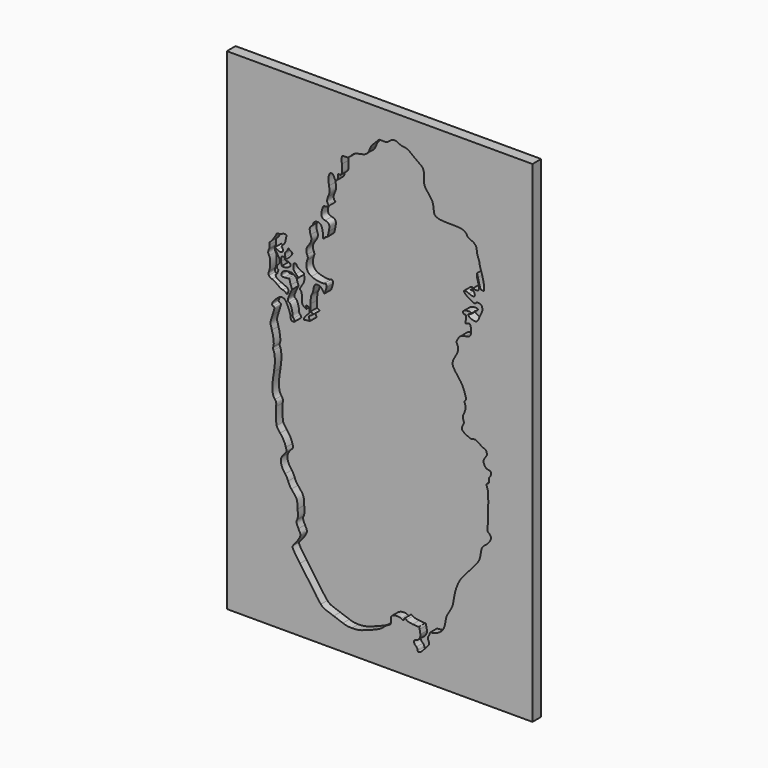
from build123d import *

# Parameters (mm, degrees)
F0_W     = 112
F0_H     = 180
F1_DEPTH = 3
F2_W     = 112
F2_H     = 180
F3_DEPTH = 1


# Not quite as in the source:
# - ends of sketch curves that miss each other by under 0.0002 mm in the source are joined


with BuildPart() as f1:
    # F0 (on Front) → F1 (new body)
    with BuildSketch(Plane.XZ):
        Rectangle(F0_W, F0_H)
        with BuildLine():
            add(Edge.make_bspline(
                [(-33.452207, 20.1281), (-33.452207, 18.937311), (-33.942265, 18.492438), (-34.505892, 19.171568)],
                knots=[0, 0, 0, 0, 1, 1, 1, 1], degree=3))
            add(Edge.make_bspline(
                [(-34.505892, 19.171568), (-34.648261, 19.343113), (-35.112361, 19.545961), (-35.537226, 19.622341)],
                knots=[0, 0, 0, 0, 1, 1, 1, 1], degree=3))
            add(Edge.make_bspline(
                [(-35.537226, 19.622341), (-35.985093, 19.702854), (-36.785926, 20.149145), (-37.44296, 20.684371)],
                knots=[0, 0, 0, 0, 1, 1, 1, 1], degree=3))
            add(Edge.make_bspline(
                [(-37.44296, 20.684371), (-38.066249, 21.192106), (-38.956872, 21.721577), (-39.42212, 21.860967)],
                knots=[0, 0, 0, 0, 1, 1, 1, 1], degree=3))
            add(Edge.make_bspline(
                [(-39.42212, 21.860967), (-39.887369, 22.00036), (-40.413552, 22.336506), (-40.591415, 22.60796)],
                knots=[0, 0, 0, 0, 1, 1, 1, 1], degree=3))
            add(Edge.make_bspline(
                [(-40.591415, 22.60796), (-40.884851, 23.055799), (-40.878115, 23.19424), (-40.518688, 24.102673)],
                knots=[0, 0, 0, 0, 1, 1, 1, 1], degree=3))
            add(Edge.make_bspline(
                [(-40.518688, 24.102673), (-39.981468, 25.46047), (-39.965306, 28.273475), (-40.490123, 29.074448)],
                knots=[0, 0, 0, 0, 1, 1, 1, 1], degree=3))
            add(Edge.make_bspline(
                [(-40.490123, 29.074448), (-40.941459, 29.763275), (-40.958652, 30.332629), (-40.551871, 31.119259)],
                knots=[0, 0, 0, 0, 1, 1, 1, 1], degree=3))
            add(Edge.make_bspline(
                [(-40.551871, 31.119259), (-40.351264, 31.507192), (-40.288878, 31.997631), (-40.373672, 32.520154)],
                knots=[0, 0, 0, 0, 1, 1, 1, 1], degree=3))
            add(Edge.make_bspline(
                [(-40.373672, 32.520154), (-40.485237, 33.207653), (-40.426908, 33.388001), (-39.97111, 33.764826)],
                knots=[0, 0, 0, 0, 1, 1, 1, 1], degree=3))
            add(Edge.make_bspline(
                [(-39.97111, 33.764826), (-39.453275, 34.19294), (-38.119119, 36.156558), (-37.838064, 36.904252)],
                knots=[0, 0, 0, 0, 1, 1, 1, 1], degree=3))
            add(Edge.make_bspline(
                [(-37.838064, 36.904252), (-37.73813, 37.170111), (-37.465273, 37.274669), (-36.871434, 37.274669)],
                knots=[0, 0, 0, 0, 1, 1, 1, 1], degree=3))
            add(Edge.make_bspline(
                [(-36.871434, 37.274669), (-36.394197, 37.274669), (-35.932527, 37.409038), (-35.78054, 37.592169)],
                knots=[0, 0, 0, 0, 1, 1, 1, 1], degree=3))
            add(Edge.make_bspline(
                [(-35.78054, 37.592169), (-35.635614, 37.766794), (-35.201315, 37.909669), (-34.81543, 37.909669)],
                knots=[0, 0, 0, 0, 1, 1, 1, 1], degree=3))
            add(Edge.make_bspline(
                [(-34.81543, 37.909669), (-34.12552, 37.909669), (-34.115723, 37.89644), (-34.227866, 37.115919)],
                knots=[0, 0, 0, 0, 1, 1, 1, 1], degree=3))
            add(Edge.make_bspline(
                [(-34.227866, 37.115919), (-34.465384, 35.462792), (-34.746487, 34.75187), (-35.370122, 34.227116)],
                knots=[0, 0, 0, 0, 1, 1, 1, 1], degree=3))
            add(Edge.make_bspline(
                [(-35.370122, 34.227116), (-35.987808, 33.707369), (-35.99809, 33.670422), (-35.666071, 33.163698)],
                knots=[0, 0, 0, 0, 1, 1, 1, 1], degree=3))
            add(Edge.make_bspline(
                [(-35.666071, 33.163698), (-34.871015, 31.950289), (-36.098201, 31.13996), (-37.504851, 31.949527)],
                knots=[0, 0, 0, 0, 1, 1, 1, 1], degree=3))
            add(Edge.make_bspline(
                [(-37.504851, 31.949527), (-37.9414, 32.200773), (-38.348154, 32.406336), (-38.408749, 32.406336)],
                knots=[0, 0, 0, 0, 1, 1, 1, 1], degree=3))
            add(Edge.make_bspline(
                [(-38.408749, 32.406336), (-38.626291, 32.406336), (-38.234714, 31.645251), (-37.438128, 30.519796)],
                knots=[0, 0, 0, 0, 1, 1, 1, 1], degree=3))
            add(Edge.make_bspline(
                [(-37.438128, 30.519796), (-36.438781, 29.10787), (-36.348556, 28.085243), (-37.156373, 27.326336)],
                knots=[0, 0, 0, 0, 1, 1, 1, 1], degree=3))
            add(Edge.make_bspline(
                [(-37.156373, 27.326336), (-37.745641, 26.772748), (-37.875697, 25.844669), (-37.364007, 25.844669)],
                knots=[0, 0, 0, 0, 1, 1, 1, 1], degree=3))
            add(Edge.make_bspline(
                [(-37.364007, 25.844669), (-37.120623, 25.844669), (-37.076294, 25.703194), (-37.181621, 25.262586)],
                knots=[0, 0, 0, 0, 1, 1, 1, 1], degree=3))
            add(Edge.make_bspline(
                [(-37.181621, 25.262586), (-37.371891, 24.46664), (-37.659904, 23.939669), (-37.904654, 23.939669)],
                knots=[0, 0, 0, 0, 1, 1, 1, 1], degree=3))
            add(Edge.make_bspline(
                [(-37.904654, 23.939669), (-38.249061, 23.939669), (-38.131257, 23.178873), (-37.730723, 22.816394)],
                knots=[0, 0, 0, 0, 1, 1, 1, 1], degree=3))
            add(Edge.make_bspline(
                [(-37.730723, 22.816394), (-37.522741, 22.628172), (-36.879803, 22.270929), (-36.301973, 22.022519)],
                knots=[0, 0, 0, 0, 1, 1, 1, 1], degree=3))
            add(Edge.make_bspline(
                [(-36.301973, 22.022519), (-33.610738, 20.865557), (-33.452207, 20.760171), (-33.452207, 20.1281)],
                knots=[0, 0, 0, 0, 1, 1, 1, 1], degree=3))
        make_face(mode=Mode.SUBTRACT)
        with BuildLine():
            add(Edge.make_bspline(
                [(-33.340422, 27.616181), (-33.616353, 27.238822), (-35.648352, 26.940163), (-35.837719, 27.249133)],
                knots=[0, 0, 0, 0, 1, 1, 1, 1], degree=3))
            add(Edge.make_bspline(
                [(-35.837719, 27.249133), (-35.89942, 27.349804), (-36.013493, 27.956044), (-36.091215, 28.596336)],
                knots=[0, 0, 0, 0, 1, 1, 1, 1], degree=3))
            add(Edge.make_bspline(
                [(-36.091215, 28.596336), (-36.274204, 30.10386), (-35.909746, 30.724602), (-35.067067, 30.340649)],
                knots=[0, 0, 0, 0, 1, 1, 1, 1], degree=3))
            add(Edge.make_bspline(
                [(-35.067067, 30.340649), (-34.706043, 30.176155), (-34.561325, 29.980284), (-34.643192, 29.766942)],
                knots=[0, 0, 0, 0, 1, 1, 1, 1], degree=3))
            add(Edge.make_bspline(
                [(-34.643192, 29.766942), (-34.738688, 29.51808), (-34.611852, 29.443002), (-34.095937, 29.443002)],
                knots=[0, 0, 0, 0, 1, 1, 1, 1], degree=3))
            add(Edge.make_bspline(
                [(-34.095937, 29.443002), (-33.144865, 29.443002), (-32.60554, 29.095631), (-32.60554, 28.483057)],
                knots=[0, 0, 0, 0, 1, 1, 1, 1], degree=3))
            add(Edge.make_bspline(
                [(-32.60554, 28.483057), (-32.60554, 28.196111), (-32.714102, 27.961336), (-32.846789, 27.961336)],
                knots=[0, 0, 0, 0, 1, 1, 1, 1], degree=3))
            add(Edge.make_bspline(
                [(-32.846789, 27.961336), (-32.979476, 27.961336), (-33.201611, 27.806015), (-33.340422, 27.616181)],
                knots=[0, 0, 0, 0, 1, 1, 1, 1], degree=3))
        make_face(mode=Mode.SUBTRACT)
        with BuildLine():
            add(Edge.make_bspline(
                [(-32.939588, 31.083419), (-34.007659, 29.963927), (-34.186452, 29.895773), (-34.503093, 30.487421)],
                knots=[0, 0, 0, 0, 1, 1, 1, 1], degree=3))
            add(Edge.make_bspline(
                [(-34.503093, 30.487421), (-34.871546, 31.175883), (-34.750485, 31.973967), (-34.19304, 32.531412)],
                knots=[0, 0, 0, 0, 1, 1, 1, 1], degree=3))
            add(Edge.make_bspline(
                [(-34.19304, 32.531412), (-33.901999, 32.822454), (-33.663874, 33.199123), (-33.663874, 33.368456)],
                knots=[0, 0, 0, 0, 1, 1, 1, 1], degree=3))
            add(Edge.make_bspline(
                [(-33.663874, 33.368456), (-33.663874, 33.537789), (-33.568624, 33.676336), (-33.452207, 33.676336)],
                knots=[0, 0, 0, 0, 1, 1, 1, 1], degree=3))
            add(Edge.make_bspline(
                [(-33.452207, 33.676336), (-33.33579, 33.676336), (-33.24054, 33.601969), (-33.24054, 33.511077)],
                knots=[0, 0, 0, 0, 1, 1, 1, 1], degree=3))
            add(Edge.make_bspline(
                [(-33.24054, 33.511077), (-33.24054, 33.420182), (-32.95479, 33.237955), (-32.60554, 33.106127)],
                knots=[0, 0, 0, 0, 1, 1, 1, 1], degree=3))
            add(Edge.make_bspline(
                [(-32.60554, 33.106127), (-31.721987, 32.772625), (-31.804468, 32.273189), (-32.939588, 31.083419)],
                knots=[0, 0, 0, 0, 1, 1, 1, 1], degree=3))
        make_face(mode=Mode.SUBTRACT)
        with BuildLine():
            add(Edge.make_bspline(
                [(-33.181515, 16.37951), (-33.856509, 16.687056), (-33.794526, 17.270613), (-32.88299, 19.190049)],
                knots=[0, 0, 0, 0, 1, 1, 1, 1], degree=3))
            Line((-32.88299, 19.190049), (-32.102106, 20.834368))
            Line((-32.102106, 20.834368), (-32.56549, 22.162106))
            add(Edge.make_bspline(
                [(-32.56549, 22.162106), (-32.820351, 22.892361), (-33.028874, 23.645098), (-33.028874, 23.834852)],
                knots=[0, 0, 0, 0, 1, 1, 1, 1], degree=3))
            add(Edge.make_bspline(
                [(-33.028874, 23.834852), (-33.028874, 24.101586), (-33.136928, 24.141533), (-33.505124, 24.010929)],
                knots=[0, 0, 0, 0, 1, 1, 1, 1], degree=3))
            add(Edge.make_bspline(
                [(-33.505124, 24.010929), (-33.767061, 23.918015), (-34.409999, 23.840159), (-34.933874, 23.837916)],
                knots=[0, 0, 0, 0, 1, 1, 1, 1], degree=3))
            add(Edge.make_bspline(
                [(-34.933874, 23.837916), (-35.841877, 23.834026), (-35.889325, 23.864003), (-35.949561, 24.479652)],
                knots=[0, 0, 0, 0, 1, 1, 1, 1], degree=3))
            add(Edge.make_bspline(
                [(-35.949561, 24.479652), (-36.054367, 25.550836), (-34.784788, 26.268002), (-32.783695, 26.268002)],
                knots=[0, 0, 0, 0, 1, 1, 1, 1], degree=3))
            add(Edge.make_bspline(
                [(-32.783695, 26.268002), (-31.934397, 26.268002), (-31.641586, 26.1596), (-31.104508, 25.646337)],
                knots=[0, 0, 0, 0, 1, 1, 1, 1], degree=3))
            add(Edge.make_bspline(
                [(-31.104508, 25.646337), (-30.746726, 25.304422), (-30.318968, 25.076488), (-30.153934, 25.139819)],
                knots=[0, 0, 0, 0, 1, 1, 1, 1], degree=3))
            add(Edge.make_bspline(
                [(-30.153934, 25.139819), (-29.704821, 25.312158), (-29.774591, 25.46967), (-30.70054, 26.373836)],
                knots=[0, 0, 0, 0, 1, 1, 1, 1], degree=3))
            add(Edge.make_bspline(
                [(-30.70054, 26.373836), (-31.495874, 27.150459), (-31.547207, 27.27498), (-31.547207, 28.427627)],
                knots=[0, 0, 0, 0, 1, 1, 1, 1], degree=3))
            add(Edge.make_bspline(
                [(-31.547207, 28.427627), (-31.547207, 29.59536), (-31.52163, 29.654669), (-31.01804, 29.654669)],
                knots=[0, 0, 0, 0, 1, 1, 1, 1], degree=3))
            add(Edge.make_bspline(
                [(-31.01804, 29.654669), (-30.703175, 29.654669), (-30.488874, 29.533506), (-30.488874, 29.355481)],
                knots=[0, 0, 0, 0, 1, 1, 1, 1], degree=3))
            add(Edge.make_bspline(
                [(-30.488874, 29.355481), (-30.488874, 28.942654), (-28.818079, 27.749669), (-28.239906, 27.749669)],
                knots=[0, 0, 0, 0, 1, 1, 1, 1], degree=3))
            add(Edge.make_bspline(
                [(-28.239906, 27.749669), (-27.826624, 27.749669), (-27.749631, 27.605302), (-27.623187, 26.593281)],
                knots=[0, 0, 0, 0, 1, 1, 1, 1], degree=3))
            add(Edge.make_bspline(
                [(-27.623187, 26.593281), (-27.456287, 25.257458), (-27.655596, 24.548041), (-28.571998, 23.216097)],
                knots=[0, 0, 0, 0, 1, 1, 1, 1], degree=3))
            add(Edge.make_bspline(
                [(-28.571998, 23.216097), (-29.211875, 22.286068), (-29.401763, 21.611336), (-29.023622, 21.611336)],
                knots=[0, 0, 0, 0, 1, 1, 1, 1], degree=3))
            add(Edge.make_bspline(
                [(-29.023622, 21.611336), (-28.661322, 21.611336), (-28.350372, 20.184647), (-28.485856, 19.143974)],
                knots=[0, 0, 0, 0, 1, 1, 1, 1], degree=3))
            add(Edge.make_bspline(
                [(-28.485856, 19.143974), (-28.655825, 17.838422), (-28.355406, 17.06631), (-27.506697, 16.627424)],
                knots=[0, 0, 0, 0, 1, 1, 1, 1], degree=3))
            Line((-27.506697, 16.627424), (-26.834667, 16.279905))
            Line((-26.834667, 16.279905), (-26.97247, 16.828955))
            add(Edge.make_bspline(
                [(-26.97247, 16.828955), (-27.09716, 17.32576), (-27.051623, 17.378002), (-26.493886, 17.378002)],
                knots=[0, 0, 0, 0, 1, 1, 1, 1], degree=3))
            add(Edge.make_bspline(
                [(-26.493886, 17.378002), (-25.814757, 17.378002), (-25.6215, 17.082016), (-25.618818, 16.037774)],
                knots=[0, 0, 0, 0, 1, 1, 1, 1], degree=3))
            add(Edge.make_bspline(
                [(-25.618818, 16.037774), (-25.617469, 15.509523), (-25.818313, 15.18744), (-26.564986, 14.520502)],
                knots=[0, 0, 0, 0, 1, 1, 1, 1], degree=3))
            add(Edge.make_bspline(
                [(-26.564986, 14.520502), (-27.088954, 14.052486), (-27.576987, 13.398825), (-27.65623, 13.05891)],
                knots=[0, 0, 0, 0, 1, 1, 1, 1], degree=3))
            add(Edge.make_bspline(
                [(-27.65623, 13.05891), (-27.789069, 12.489095), (-27.762358, 12.453945), (-27.292147, 12.57977)],
                knots=[0, 0, 0, 0, 1, 1, 1, 1], degree=3))
            add(Edge.make_bspline(
                [(-27.292147, 12.57977), (-27.013055, 12.654452), (-26.471793, 12.716856), (-26.089343, 12.718446)],
                knots=[0, 0, 0, 0, 1, 1, 1, 1], degree=3))
            add(Edge.make_bspline(
                [(-26.089343, 12.718446), (-25.467765, 12.721092), (-25.41723, 12.764778), (-25.613093, 13.130755)],
                knots=[0, 0, 0, 0, 1, 1, 1, 1], degree=3))
            add(Edge.make_bspline(
                [(-25.613093, 13.130755), (-26.016484, 13.884497), (-25.882158, 14.605735), (-25.311723, 14.748904)],
                knots=[0, 0, 0, 0, 1, 1, 1, 1], degree=3))
            add(Edge.make_bspline(
                [(-25.311723, 14.748904), (-25.025456, 14.820751), (-24.681728, 15.01149), (-24.547883, 15.172761)],
                knots=[0, 0, 0, 0, 1, 1, 1, 1], degree=3))
            add(Edge.make_bspline(
                [(-24.547883, 15.172761), (-24.354366, 15.405936), (-24.416942, 15.508726), (-24.85344, 15.674684)],
                knots=[0, 0, 0, 0, 1, 1, 1, 1], degree=3))
            Line((-24.85344, 15.674684), (-25.402351, 15.883379))
            Line((-25.402351, 15.883379), (-25.337298, 18.401704))
            add(Edge.make_bspline(
                [(-25.337298, 18.401704), (-25.283362, 20.489637), (-25.197538, 21.046649), (-24.835122, 21.660895)],
                knots=[0, 0, 0, 0, 1, 1, 1, 1], degree=3))
            add(Edge.make_bspline(
                [(-24.835122, 21.660895), (-24.594705, 22.068374), (-24.329432, 22.91448), (-24.245626, 23.541132)],
                knots=[0, 0, 0, 0, 1, 1, 1, 1], degree=3))
            add(Edge.make_bspline(
                [(-24.245626, 23.541132), (-24.053642, 24.976677), (-23.674132, 25.421336), (-22.640895, 25.421336)],
                knots=[0, 0, 0, 0, 1, 1, 1, 1], degree=3))
            add(Edge.make_bspline(
                [(-22.640895, 25.421336), (-21.966808, 25.421336), (-21.726439, 25.284546), (-21.086201, 24.536569)],
                knots=[0, 0, 0, 0, 1, 1, 1, 1], degree=3))
            add(Edge.make_bspline(
                [(-21.086201, 24.536569), (-20.669671, 24.049947), (-20.323552, 23.549885), (-20.317048, 23.425319)],
                knots=[0, 0, 0, 0, 1, 1, 1, 1], degree=3))
            add(Edge.make_bspline(
                [(-20.317048, 23.425319), (-20.291121, 22.928799), (-19.505283, 25.146547), (-19.497276, 25.738836)],
                knots=[0, 0, 0, 0, 1, 1, 1, 1], degree=3))
            add(Edge.make_bspline(
                [(-19.497276, 25.738836), (-19.484513, 26.683165), (-19.747962, 27.005002), (-20.267936, 26.680271)],
                knots=[0, 0, 0, 0, 1, 1, 1, 1], degree=3))
            add(Edge.make_bspline(
                [(-20.267936, 26.680271), (-20.841746, 26.321922), (-23.700708, 26.748536), (-24.985541, 27.384234)],
                knots=[0, 0, 0, 0, 1, 1, 1, 1], degree=3))
            add(Edge.make_bspline(
                [(-24.985541, 27.384234), (-26.691258, 28.228173), (-27.267401, 29.9549), (-26.547871, 32.066603)],
                knots=[0, 0, 0, 0, 1, 1, 1, 1], degree=3))
            add(Edge.make_bspline(
                [(-26.547871, 32.066603), (-26.227972, 33.005458), (-26.22989, 33.127032), (-26.576744, 33.896215)],
                knots=[0, 0, 0, 0, 1, 1, 1, 1], degree=3))
            add(Edge.make_bspline(
                [(-26.576744, 33.896215), (-27.035529, 34.91362), (-26.897942, 35.994083), (-26.191194, 36.923929)],
                knots=[0, 0, 0, 0, 1, 1, 1, 1], degree=3))
            add(Edge.make_bspline(
                [(-26.191194, 36.923929), (-24.961255, 38.542121), (-24.755625, 39.424372), (-25.303041, 40.734522)],
                knots=[0, 0, 0, 0, 1, 1, 1, 1], degree=3))
            add(Edge.make_bspline(
                [(-25.303041, 40.734522), (-25.477666, 41.152458), (-25.620541, 41.871979), (-25.620541, 42.33346)],
                knots=[0, 0, 0, 0, 1, 1, 1, 1], degree=3))
            add(Edge.make_bspline(
                [(-25.620541, 42.33346), (-25.620541, 43.024147), (-25.508258, 43.252464), (-24.985541, 43.624672)],
                knots=[0, 0, 0, 0, 1, 1, 1, 1], degree=3))
            add(Edge.make_bspline(
                [(-24.985541, 43.624672), (-24.636291, 43.873359), (-24.350541, 44.257134), (-24.350541, 44.477506)],
                knots=[0, 0, 0, 0, 1, 1, 1, 1], degree=3))
            add(Edge.make_bspline(
                [(-24.350541, 44.477506), (-24.350541, 45.594248), (-22.431199, 46.16264), (-21.615768, 45.287374)],
                knots=[0, 0, 0, 0, 1, 1, 1, 1], degree=3))
            add(Edge.make_bspline(
                [(-21.615768, 45.287374), (-21.109145, 44.743579), (-20.662783, 42.776066), (-20.822605, 41.791199)],
                knots=[0, 0, 0, 0, 1, 1, 1, 1], degree=3))
            add(Edge.make_bspline(
                [(-20.822605, 41.791199), (-20.954781, 40.976693), (-20.499399, 40.793873), (-20.117207, 41.508005)],
                knots=[0, 0, 0, 0, 1, 1, 1, 1], degree=3))
            add(Edge.make_bspline(
                [(-20.117207, 41.508005), (-19.992599, 41.740838), (-19.705312, 41.931338), (-19.478793, 41.931338)],
                knots=[0, 0, 0, 0, 1, 1, 1, 1], degree=3))
            add(Edge.make_bspline(
                [(-19.478793, 41.931338), (-19.198062, 41.931338), (-19.030888, 42.116655), (-18.953701, 42.513422)],
                knots=[0, 0, 0, 0, 1, 1, 1, 1], degree=3))
            add(Edge.make_bspline(
                [(-18.953701, 42.513422), (-18.89142, 42.833567), (-18.746731, 43.501683), (-18.632169, 43.998126)],
                knots=[0, 0, 0, 0, 1, 1, 1, 1], degree=3))
            add(Edge.make_bspline(
                [(-18.632169, 43.998126), (-18.149076, 46.091551), (-18.464465, 46.832284), (-19.952374, 47.09881)],
                knots=[0, 0, 0, 0, 1, 1, 1, 1], degree=3))
            add(Edge.make_bspline(
                [(-19.952374, 47.09881), (-21.372442, 47.353185), (-21.67856, 48.313191), (-21.020685, 50.449112)],
                knots=[0, 0, 0, 0, 1, 1, 1, 1], degree=3))
            add(Edge.make_bspline(
                [(-21.020685, 50.449112), (-20.672024, 51.581108), (-20.602006, 51.66451), (-19.998913, 51.666195)],
                knots=[0, 0, 0, 0, 1, 1, 1, 1], degree=3))
            add(Edge.make_bspline(
                [(-19.998913, 51.666195), (-19.64281, 51.667254), (-19.167823, 51.802276), (-18.943389, 51.966386)],
                knots=[0, 0, 0, 0, 1, 1, 1, 1], degree=3))
            add(Edge.make_bspline(
                [(-18.943389, 51.966386), (-18.555059, 52.250342), (-18.553103, 52.28441), (-18.902935, 52.670969)],
                knots=[0, 0, 0, 0, 1, 1, 1, 1], degree=3))
            add(Edge.make_bspline(
                [(-18.902935, 52.670969), (-19.361289, 53.177445), (-19.371368, 53.987205), (-18.932029, 55.008553)],
                knots=[0, 0, 0, 0, 1, 1, 1, 1], degree=3))
            add(Edge.make_bspline(
                [(-18.932029, 55.008553), (-18.259801, 56.571305), (-18.220416, 56.95618), (-18.553202, 58.71048)],
                knots=[0, 0, 0, 0, 1, 1, 1, 1], degree=3))
            add(Edge.make_bspline(
                [(-18.553202, 58.71048), (-19.053729, 61.349042), (-18.663629, 63.098004), (-17.574581, 63.098004)],
                knots=[0, 0, 0, 0, 1, 1, 1, 1], degree=3))
            add(Edge.make_bspline(
                [(-17.574581, 63.098004), (-17.130381, 63.098004), (-16.932486, 62.855999), (-16.624707, 61.936416)],
                knots=[0, 0, 0, 0, 1, 1, 1, 1], degree=3))
            add(Edge.make_bspline(
                [(-16.624707, 61.936416), (-16.185222, 60.623311), (-15.248874, 61.364218), (-15.248874, 63.025077)],
                knots=[0, 0, 0, 0, 1, 1, 1, 1], degree=3))
            add(Edge.make_bspline(
                [(-15.248874, 63.025077), (-15.248874, 63.724734), (-15.210609, 63.769293), (-14.716325, 63.645236)],
                knots=[0, 0, 0, 0, 1, 1, 1, 1], degree=3))
            add(Edge.make_bspline(
                [(-14.716325, 63.645236), (-13.8828, 63.436035), (-13.698338, 64.212786), (-13.859917, 67.251448)],
                knots=[0, 0, 0, 0, 1, 1, 1, 1], degree=3))
            add(Edge.make_bspline(
                [(-13.859917, 67.251448), (-14.013915, 70.147494), (-14.056947, 70.07356), (-12.213489, 70.080114)],
                knots=[0, 0, 0, 0, 1, 1, 1, 1], degree=3))
            add(Edge.make_bspline(
                [(-12.213489, 70.080114), (-11.518957, 70.082575), (-11.254887, 70.234186), (-10.399825, 71.12133)],
                knots=[0, 0, 0, 0, 1, 1, 1, 1], degree=3))
            add(Edge.make_bspline(
                [(-10.399825, 71.12133), (-9.375891, 72.183684), (-9.027265, 72.337554), (-6.515171, 72.835877)],
                knots=[0, 0, 0, 0, 1, 1, 1, 1], degree=3))
            add(Edge.make_bspline(
                [(-6.515171, 72.835877), (-4.934002, 73.149533), (-4.211332, 73.775078), (-3.703224, 75.269907)],
                knots=[0, 0, 0, 0, 1, 1, 1, 1], degree=3))
            add(Edge.make_bspline(
                [(-3.703224, 75.269907), (-3.384936, 76.206291), (-2.963105, 76.802249), (-1.745516, 78.035737)],
                knots=[0, 0, 0, 0, 1, 1, 1, 1], degree=3))
            Line((-1.745516, 78.035737), (-0.193515, 79.608005))
            Line((-0.193515, 79.608005), (1.274028, 79.608005))
            add(Edge.make_bspline(
                [(1.274028, 79.608005), (2.657944, 79.608005), (2.788984, 79.650838), (3.573572, 80.359667)],
                knots=[0, 0, 0, 0, 1, 1, 1, 1], degree=3))
            add(Edge.make_bspline(
                [(3.573572, 80.359667), (4.717466, 81.393106), (5.622754, 81.514468), (6.844933, 80.798222)],
                knots=[0, 0, 0, 0, 1, 1, 1, 1], degree=3))
            add(Edge.make_bspline(
                [(6.844933, 80.798222), (7.393068, 80.476995), (8.113838, 80.243005), (8.5552, 80.243005)],
                knots=[0, 0, 0, 0, 1, 1, 1, 1], degree=3))
            add(Edge.make_bspline(
                [(8.5552, 80.243005), (9.646529, 80.243005), (10.657992, 79.759654), (12.025824, 78.584484)],
                knots=[0, 0, 0, 0, 1, 1, 1, 1], degree=3))
            add(Edge.make_bspline(
                [(12.025824, 78.584484), (12.682782, 78.020062), (13.763409, 77.213935), (14.427222, 76.793091)],
                knots=[0, 0, 0, 0, 1, 1, 1, 1], degree=3))
            add(Edge.make_bspline(
                [(14.427222, 76.793091), (16.074841, 75.748531), (16.306735, 75.227319), (16.257758, 72.678687)],
                knots=[0, 0, 0, 0, 1, 1, 1, 1], degree=3))
            add(Edge.make_bspline(
                [(16.257758, 72.678687), (16.212196, 70.307789), (16.302787, 70.061232), (17.989212, 67.966338)],
                knots=[0, 0, 0, 0, 1, 1, 1, 1], degree=3))
            add(Edge.make_bspline(
                [(17.989212, 67.966338), (19.344001, 66.283404), (19.583327, 65.731341), (19.778539, 63.838838)],
                knots=[0, 0, 0, 0, 1, 1, 1, 1], degree=3))
            add(Edge.make_bspline(
                [(19.778539, 63.838838), (19.970981, 61.973202), (20.093107, 61.754361), (21.204535, 61.283582)],
                knots=[0, 0, 0, 0, 1, 1, 1, 1], degree=3))
            add(Edge.make_bspline(
                [(21.204535, 61.283582), (21.954454, 60.965929), (22.770757, 60.893977), (25.949027, 60.865383)],
                knots=[0, 0, 0, 0, 1, 1, 1, 1], degree=3))
            add(Edge.make_bspline(
                [(25.949027, 60.865383), (29.468866, 60.833716), (29.870316, 60.790883), (30.781501, 60.349786)],
                knots=[0, 0, 0, 0, 1, 1, 1, 1], degree=3))
            add(Edge.make_bspline(
                [(30.781501, 60.349786), (31.328057, 60.085202), (31.822063, 59.71425), (31.879287, 59.525448)],
                knots=[0, 0, 0, 0, 1, 1, 1, 1], degree=3))
            add(Edge.make_bspline(
                [(31.879287, 59.525448), (32.104106, 58.783721), (32.322853, 58.58271), (33.33577, 58.18706)],
                knots=[0, 0, 0, 0, 1, 1, 1, 1], degree=3))
            add(Edge.make_bspline(
                [(33.33577, 58.18706), (34.993647, 57.539487), (35.470177, 56.959313), (35.614613, 55.412567)],
                knots=[0, 0, 0, 0, 1, 1, 1, 1], degree=3))
            add(Edge.make_bspline(
                [(35.614613, 55.412567), (35.682043, 54.690491), (35.931375, 53.671631), (36.168685, 53.148436)],
                knots=[0, 0, 0, 0, 1, 1, 1, 1], degree=3))
            add(Edge.make_bspline(
                [(36.168685, 53.148436), (36.405998, 52.625241), (36.602253, 51.938806), (36.604809, 51.623026)],
                knots=[0, 0, 0, 0, 1, 1, 1, 1], degree=3))
            add(Edge.make_bspline(
                [(36.604809, 51.623026), (36.607454, 51.307248), (36.794766, 50.545248), (37.02126, 49.929692)],
                knots=[0, 0, 0, 0, 1, 1, 1, 1], degree=3))
            add(Edge.make_bspline(
                [(37.02126, 49.929692), (37.701472, 48.081012), (38.302791, 45.422529), (38.302791, 44.26391)],
                knots=[0, 0, 0, 0, 1, 1, 1, 1], degree=3))
            Line((38.302791, 44.26391), (38.302791, 43.174515))
            Line((38.302791, 43.174515), (37.620719, 43.240843))
            add(Edge.make_bspline(
                [(37.620719, 43.240843), (36.865548, 43.314278), (36.860634, 43.325745), (36.050819, 46.905505)],
                knots=[0, 0, 0, 0, 1, 1, 1, 1], degree=3))
            add(Edge.make_bspline(
                [(36.050819, 46.905505), (35.750316, 48.233861), (35.652496, 48.453323), (35.596982, 47.923717)],
                knots=[0, 0, 0, 0, 1, 1, 1, 1], degree=3))
            add(Edge.make_bspline(
                [(35.596982, 47.923717), (35.558059, 47.552398), (35.722315, 46.613677), (35.962001, 45.837668)],
                knots=[0, 0, 0, 0, 1, 1, 1, 1], degree=3))
            add(Edge.make_bspline(
                [(35.962001, 45.837668), (36.201687, 45.061661), (36.397791, 44.158818), (36.397791, 43.831354)],
                knots=[0, 0, 0, 0, 1, 1, 1, 1], degree=3))
            add(Edge.make_bspline(
                [(36.397791, 43.831354), (36.397791, 42.724144), (36.228383, 42.566338), (35.039766, 42.566338)],
                knots=[0, 0, 0, 0, 1, 1, 1, 1], degree=3))
            add(Edge.make_bspline(
                [(35.039766, 42.566338), (34.354088, 42.566338), (33.783697, 42.440828), (33.527829, 42.233651)],
                knots=[0, 0, 0, 0, 1, 1, 1, 1], degree=3))
            add(Edge.make_bspline(
                [(33.527829, 42.233651), (33.137129, 41.917297), (33.149665, 41.906433), (33.783183, 42.012354)],
                knots=[0, 0, 0, 0, 1, 1, 1, 1], degree=3))
            add(Edge.make_bspline(
                [(33.783183, 42.012354), (34.367045, 42.109974), (34.481239, 42.046903), (34.706873, 41.502176)],
                knots=[0, 0, 0, 0, 1, 1, 1, 1], degree=3))
            add(Edge.make_bspline(
                [(34.706873, 41.502176), (35.23492, 40.22735), (34.460601, 39.889403), (32.769655, 40.65669)],
                knots=[0, 0, 0, 0, 1, 1, 1, 1], degree=3))
            add(Edge.make_bspline(
                [(32.769655, 40.65669), (29.998089, 41.91432), (30.46157, 40.257351), (33.297202, 38.770695)],
                knots=[0, 0, 0, 0, 1, 1, 1, 1], degree=3))
            add(Edge.make_bspline(
                [(33.297202, 38.770695), (34.690344, 38.040299), (35.028802, 37.981405), (35.204335, 38.438836)],
                knots=[0, 0, 0, 0, 1, 1, 1, 1], degree=3))
            add(Edge.make_bspline(
                [(35.204335, 38.438836), (35.406691, 38.966166), (36.938718, 38.856372), (37.338289, 38.285906)],
                knots=[0, 0, 0, 0, 1, 1, 1, 1], degree=3))
            add(Edge.make_bspline(
                [(37.338289, 38.285906), (37.791523, 37.638823), (37.7511, 36.506933), (37.245542, 35.688926)],
                knots=[0, 0, 0, 0, 1, 1, 1, 1], degree=3))
            add(Edge.make_bspline(
                [(37.245542, 35.688926), (37.013307, 35.313162), (36.677424, 34.59227), (36.499137, 34.08695)],
                knots=[0, 0, 0, 0, 1, 1, 1, 1], degree=3))
            add(Edge.make_bspline(
                [(36.499137, 34.08695), (36.069821, 32.870142), (35.618122, 32.406336), (34.86239, 32.406336)],
                knots=[0, 0, 0, 0, 1, 1, 1, 1], degree=3))
            add(Edge.make_bspline(
                [(34.86239, 32.406336), (34.05989, 32.406336), (32.845161, 32.983765), (32.571344, 33.495403)],
                knots=[0, 0, 0, 0, 1, 1, 1, 1], degree=3))
            add(Edge.make_bspline(
                [(32.571344, 33.495403), (32.354717, 33.900173), (32.369877, 33.913556), (33.399143, 34.22592)],
                knots=[0, 0, 0, 0, 1, 1, 1, 1], degree=3))
            add(Edge.make_bspline(
                [(33.399143, 34.22592), (33.554343, 34.273024), (33.642232, 34.430573), (33.594448, 34.576033)],
                knots=[0, 0, 0, 0, 1, 1, 1, 1], degree=3))
            add(Edge.make_bspline(
                [(33.594448, 34.576033), (33.46648, 34.965576), (32.104778, 35.015522), (31.25804, 34.661731)],
                knots=[0, 0, 0, 0, 1, 1, 1, 1], degree=3))
            add(Edge.make_bspline(
                [(31.25804, 34.661731), (30.627017, 34.398074), (30.536886, 34.274421), (30.628062, 33.797465)],
                knots=[0, 0, 0, 0, 1, 1, 1, 1], degree=3))
            add(Edge.make_bspline(
                [(30.628062, 33.797465), (30.71026, 33.367474), (30.825113, 33.269647), (31.133003, 33.367366)],
                knots=[0, 0, 0, 0, 1, 1, 1, 1], degree=3))
            add(Edge.make_bspline(
                [(31.133003, 33.367366), (31.684157, 33.542298), (31.793453, 33.125915), (31.570156, 31.701965)],
                knots=[0, 0, 0, 0, 1, 1, 1, 1], degree=3))
            add(Edge.make_bspline(
                [(31.570156, 31.701965), (31.466603, 31.04162), (31.40345, 30.501336), (31.429818, 30.501336)],
                knots=[0, 0, 0, 0, 1, 1, 1, 1], degree=3))
            add(Edge.make_bspline(
                [(31.429818, 30.501336), (31.456197, 30.501336), (31.82438, 30.646166), (32.248031, 30.823175)],
                knots=[0, 0, 0, 0, 1, 1, 1, 1], degree=3))
            add(Edge.make_bspline(
                [(32.248031, 30.823175), (33.013098, 31.142844), (33.019921, 31.141056), (33.258078, 30.558591)],
                knots=[0, 0, 0, 0, 1, 1, 1, 1], degree=3))
            add(Edge.make_bspline(
                [(33.258078, 30.558591), (33.389954, 30.236062), (33.507403, 29.432385), (33.519071, 28.772646)],
                knots=[0, 0, 0, 0, 1, 1, 1, 1], degree=3))
            add(Edge.make_bspline(
                [(33.519071, 28.772646), (33.547924, 27.141596), (33.029259, 26.568701), (31.401537, 26.433716)],
                knots=[0, 0, 0, 0, 1, 1, 1, 1], degree=3))
            add(Edge.make_bspline(
                [(31.401537, 26.433716), (29.985315, 26.316273), (29.274292, 25.826177), (28.589444, 24.495389)],
                knots=[0, 0, 0, 0, 1, 1, 1, 1], degree=3))
            add(Edge.make_bspline(
                [(28.589444, 24.495389), (28.089736, 23.524366), (28.087514, 23.495193), (28.460479, 22.802646)],
                knots=[0, 0, 0, 0, 1, 1, 1, 1], degree=3))
            add(Edge.make_bspline(
                [(28.460479, 22.802646), (29.022483, 21.759066), (28.804731, 20.502094), (27.762614, 18.774246)],
                knots=[0, 0, 0, 0, 1, 1, 1, 1], degree=3))
            add(Edge.make_bspline(
                [(27.762614, 18.774246), (26.256489, 16.27705), (26.340499, 15.601759), (28.494726, 12.889648)],
                knots=[0, 0, 0, 0, 1, 1, 1, 1], degree=3))
            add(Edge.make_bspline(
                [(28.494726, 12.889648), (30.072807, 10.902891), (30.643966, 9.852207), (31.320466, 7.691522)],
                knots=[0, 0, 0, 0, 1, 1, 1, 1], degree=3))
            add(Edge.make_bspline(
                [(31.320466, 7.691522), (31.787826, 6.198811), (31.790546, 6.141781), (31.414213, 5.725935)],
                knots=[0, 0, 0, 0, 1, 1, 1, 1], degree=3))
            add(Edge.make_bspline(
                [(31.414213, 5.725935), (31.080113, 5.356759), (31.061322, 5.201719), (31.278045, 4.602387)],
                knots=[0, 0, 0, 0, 1, 1, 1, 1], degree=3))
            add(Edge.make_bspline(
                [(31.278045, 4.602387), (31.649494, 3.575158), (31.589113, 2.919962), (31.000291, 1.588532)],
                knots=[0, 0, 0, 0, 1, 1, 1, 1], degree=3))
            add(Edge.make_bspline(
                [(31.000291, 1.588532), (30.396784, 0.223895), (30.373416, 0.004098), (30.727693, -0.975633)],
                knots=[0, 0, 0, 0, 1, 1, 1, 1], degree=3))
            add(Edge.make_bspline(
                [(30.727693, -0.975633), (30.955542, -1.605743), (30.927311, -1.789409), (30.475447, -2.616587)],
                knots=[0, 0, 0, 0, 1, 1, 1, 1], degree=3))
            add(Edge.make_bspline(
                [(30.475447, -2.616587), (29.7633, -3.920231), (30.025357, -4.405525), (31.970409, -5.385036)],
                knots=[0, 0, 0, 0, 1, 1, 1, 1], degree=3))
            add(Edge.make_bspline(
                [(31.970409, -5.385036), (33.321475, -6.065422), (33.549887, -6.120543), (34.090428, -5.896645)],
                knots=[0, 0, 0, 0, 1, 1, 1, 1], degree=3))
            add(Edge.make_bspline(
                [(34.090428, -5.896645), (34.889285, -5.565749), (35.482369, -5.737696), (36.669999, -6.644519)],
                knots=[0, 0, 0, 0, 1, 1, 1, 1], degree=3))
            add(Edge.make_bspline(
                [(36.669999, -6.644519), (37.210189, -7.056983), (37.935872, -7.451199), (38.282632, -7.520549)],
                knots=[0, 0, 0, 0, 1, 1, 1, 1], degree=3))
            add(Edge.make_bspline(
                [(38.282632, -7.520549), (38.740107, -7.612044), (38.97457, -7.822968), (39.137112, -8.28924)],
                knots=[0, 0, 0, 0, 1, 1, 1, 1], degree=3))
            add(Edge.make_bspline(
                [(39.137112, -8.28924), (39.460068, -9.215668), (39.429982, -9.35881), (38.726124, -10.244498)],
                knots=[0, 0, 0, 0, 1, 1, 1, 1], degree=3))
            add(Edge.make_bspline(
                [(38.726124, -10.244498), (37.951628, -11.219075), (37.90378, -12.125429), (38.574131, -13.123614)],
                knots=[0, 0, 0, 0, 1, 1, 1, 1], degree=3))
            add(Edge.make_bspline(
                [(38.574131, -13.123614), (38.940865, -13.669698), (39.233402, -13.859714), (39.789363, -13.912967)],
                knots=[0, 0, 0, 0, 1, 1, 1, 1], degree=3))
            add(Edge.make_bspline(
                [(39.789363, -13.912967), (40.19209, -13.951543), (40.592402, -14.094418), (40.67895, -14.230467)],
                knots=[0, 0, 0, 0, 1, 1, 1, 1], degree=3))
            add(Edge.make_bspline(
                [(40.67895, -14.230467), (40.980395, -14.704333), (40.839756, -15.579133), (40.397833, -15.979069)],
                knots=[0, 0, 0, 0, 1, 1, 1, 1], degree=3))
            add(Edge.make_bspline(
                [(40.397833, -15.979069), (40.041643, -16.301416), (39.972642, -16.557123), (40.051959, -17.260824)],
                knots=[0, 0, 0, 0, 1, 1, 1, 1], degree=3))
            add(Edge.make_bspline(
                [(40.051959, -17.260824), (40.138488, -18.028508), (40.087588, -18.168816), (39.65025, -18.368079)],
                knots=[0, 0, 0, 0, 1, 1, 1, 1], degree=3))
            add(Edge.make_bspline(
                [(39.65025, -18.368079), (39.058729, -18.637594), (39.032609, -18.909729), (39.492834, -20.008234)],
                knots=[0, 0, 0, 0, 1, 1, 1, 1], degree=3))
            add(Edge.make_bspline(
                [(39.492834, -20.008234), (39.770995, -20.672171), (39.831842, -21.57153), (39.813212, -24.743664)],
                knots=[0, 0, 0, 0, 1, 1, 1, 1], degree=3))
            add(Edge.make_bspline(
                [(39.813212, -24.743664), (39.800565, -26.897373), (39.72854, -29.823717), (39.653166, -31.246649)],
                knots=[0, 0, 0, 0, 1, 1, 1, 1], degree=3))
            Line((39.653166, -31.246649), (39.516117, -33.8338))
            Line((39.516117, -33.8338), (40.179454, -34.415868))
            add(Edge.make_bspline(
                [(40.179454, -34.415868), (40.54429, -34.736003), (40.842791, -35.184776), (40.842791, -35.413138)],
                knots=[0, 0, 0, 0, 1, 1, 1, 1], degree=3))
            add(Edge.make_bspline(
                [(40.842791, -35.413138), (40.842791, -36.269541), (39.95722, -37.647838), (38.915772, -38.412328)],
                knots=[0, 0, 0, 0, 1, 1, 1, 1], degree=3))
            add(Edge.make_bspline(
                [(38.915772, -38.412328), (37.625246, -39.35966), (37.284899, -39.992486), (37.047015, -41.886995)],
                knots=[0, 0, 0, 0, 1, 1, 1, 1], degree=3))
            add(Edge.make_bspline(
                [(37.047015, -41.886995), (36.944936, -42.699959), (36.663221, -43.77453), (36.420981, -44.274928)],
                knots=[0, 0, 0, 0, 1, 1, 1, 1], degree=3))
            add(Edge.make_bspline(
                [(36.420981, -44.274928), (35.963088, -45.220806), (33.779575, -47.874484), (31.291028, -50.50948)],
                knots=[0, 0, 0, 0, 1, 1, 1, 1], degree=3))
            add(Edge.make_bspline(
                [(31.291028, -50.50948), (29.016167, -52.918215), (27.805145, -55.657346), (27.194778, -59.7745)],
                knots=[0, 0, 0, 0, 1, 1, 1, 1], degree=3))
            add(Edge.make_bspline(
                [(27.194778, -59.7745), (26.845033, -62.133681), (26.75259, -62.36852), (25.139955, -64.994565)],
                knots=[0, 0, 0, 0, 1, 1, 1, 1], degree=3))
            add(Edge.make_bspline(
                [(25.139955, -64.994565), (24.575392, -65.913908), (24.347724, -66.591077), (24.162248, -67.902622)],
                knots=[0, 0, 0, 0, 1, 1, 1, 1], degree=3))
            add(Edge.make_bspline(
                [(24.162248, -67.902622), (23.875577, -69.92974), (23.3596, -71.034857), (22.28704, -71.918952)],
                knots=[0, 0, 0, 0, 1, 1, 1, 1], degree=3))
            add(Edge.make_bspline(
                [(22.28704, -71.918952), (21.42521, -72.629345), (19.940951, -73.215334), (19.003418, -73.215334)],
                knots=[0, 0, 0, 0, 1, 1, 1, 1], degree=3))
            add(Edge.make_bspline(
                [(19.003418, -73.215334), (18.592134, -73.215334), (18.406124, -73.322908), (18.406124, -73.560768)],
                knots=[0, 0, 0, 0, 1, 1, 1, 1], degree=3))
            add(Edge.make_bspline(
                [(18.406124, -73.560768), (18.406124, -73.750755), (18.211727, -74.22074), (17.974134, -74.605177)],
                knots=[0, 0, 0, 0, 1, 1, 1, 1], degree=3))
            add(Edge.make_bspline(
                [(17.974134, -74.605177), (17.569138, -75.26047), (17.562524, -75.352939), (17.8683, -76.084758)],
                knots=[0, 0, 0, 0, 1, 1, 1, 1], degree=3))
            add(Edge.make_bspline(
                [(17.8683, -76.084758), (18.344542, -77.224568), (18.298642, -77.382516), (17.142961, -78.580856)],
                knots=[0, 0, 0, 0, 1, 1, 1, 1], degree=3))
            add(Edge.make_bspline(
                [(17.142961, -78.580856), (16.56464, -79.180529), (15.874077, -79.929519), (15.608378, -80.245281)],
                knots=[0, 0, 0, 0, 1, 1, 1, 1], degree=3))
            add(Edge.make_bspline(
                [(15.608378, -80.245281), (15.342683, -80.561043), (14.863353, -80.880932), (14.543207, -80.956145)],
                knots=[0, 0, 0, 0, 1, 1, 1, 1], degree=3))
            add(Edge.make_bspline(
                [(14.543207, -80.956145), (14.025285, -81.077819), (13.961124, -81.033729), (13.961124, -80.556143)],
                knots=[0, 0, 0, 0, 1, 1, 1, 1], degree=3))
            add(Edge.make_bspline(
                [(13.961124, -80.556143), (13.961124, -80.245427), (13.752439, -79.85524), (13.465573, -79.62959)],
                knots=[0, 0, 0, 0, 1, 1, 1, 1], degree=3))
            add(Edge.make_bspline(
                [(13.465573, -79.62959), (12.326835, -78.733859), (12.309648, -77.448667), (13.436402, -77.448667)],
                knots=[0, 0, 0, 0, 1, 1, 1, 1], degree=3))
            add(Edge.make_bspline(
                [(13.436402, -77.448667), (14.202395, -77.448667), (15.114221, -76.006892), (14.939172, -75.072492)],
                knots=[0, 0, 0, 0, 1, 1, 1, 1], degree=3))
            add(Edge.make_bspline(
                [(14.939172, -75.072492), (14.867766, -74.691346), (14.748143, -74.017198), (14.67334, -73.574384)],
                knots=[0, 0, 0, 0, 1, 1, 1, 1], degree=3))
            add(Edge.make_bspline(
                [(14.67334, -73.574384), (14.579416, -73.018373), (14.448793, -72.803245), (14.25116, -72.879083)],
                knots=[0, 0, 0, 0, 1, 1, 1, 1], degree=3))
            add(Edge.make_bspline(
                [(14.25116, -72.879083), (14.093765, -72.939482), (13.130682, -72.884718), (12.110972, -72.757364)],
                knots=[0, 0, 0, 0, 1, 1, 1, 1], degree=3))
            add(Edge.make_bspline(
                [(12.110972, -72.757364), (10.798538, -72.593465), (10.122417, -72.403653), (9.796379, -72.107574)],
                knots=[0, 0, 0, 0, 1, 1, 1, 1], degree=3))
            add(Edge.make_bspline(
                [(9.796379, -72.107574), (9.316239, -71.671553), (8.881124, -71.751301), (8.881124, -72.275325)],
                knots=[0, 0, 0, 0, 1, 1, 1, 1], degree=3))
            add(Edge.make_bspline(
                [(8.881124, -72.275325), (8.881124, -72.657862), (8.50608, -72.653435), (7.822791, -72.262836)],
                knots=[0, 0, 0, 0, 1, 1, 1, 1], degree=3))
            add(Edge.make_bspline(
                [(7.822791, -72.262836), (7.113734, -71.857505), (5.826639, -71.868287), (4.944365, -72.286966)],
                knots=[0, 0, 0, 0, 1, 1, 1, 1], degree=3))
            add(Edge.make_bspline(
                [(4.944365, -72.286966), (4.155155, -72.661468), (4.175274, -72.611655), (4.14196, -74.273683)],
                knots=[0, 0, 0, 0, 1, 1, 1, 1], degree=3))
            add(Edge.make_bspline(
                [(4.14196, -74.273683), (4.11873, -75.432248), (4.114081, -75.440141), (3.174083, -75.914152)],
                knots=[0, 0, 0, 0, 1, 1, 1, 1], degree=3))
            add(Edge.make_bspline(
                [(3.174083, -75.914152), (2.654584, -76.176122), (1.838212, -76.774514), (1.359922, -77.243919)],
                knots=[0, 0, 0, 0, 1, 1, 1, 1], degree=3))
            add(Edge.make_bspline(
                [(1.359922, -77.243919), (0.677011, -77.914148), (-0.188129, -78.371602), (-2.669701, -79.374648)],
                knots=[0, 0, 0, 0, 1, 1, 1, 1], degree=3))
            add(Edge.make_bspline(
                [(-2.669701, -79.374648), (-6.494255, -80.920519), (-7.822337, -81.25283), (-10.168873, -81.251089)],
                knots=[0, 0, 0, 0, 1, 1, 1, 1], degree=3))
            add(Edge.make_bspline(
                [(-10.168873, -81.251089), (-11.588961, -81.250031), (-12.280225, -81.13299), (-13.449707, -80.695578)],
                knots=[0, 0, 0, 0, 1, 1, 1, 1], degree=3))
            add(Edge.make_bspline(
                [(-13.449707, -80.695578), (-14.264623, -80.390768), (-15.788624, -79.85864), (-16.836374, -79.513057)],
                knots=[0, 0, 0, 0, 1, 1, 1, 1], degree=3))
            add(Edge.make_bspline(
                [(-16.836374, -79.513057), (-20.425463, -78.329253), (-20.59072, -78.250251), (-21.54897, -77.260162)],
                knots=[0, 0, 0, 0, 1, 1, 1, 1], degree=3))
            add(Edge.make_bspline(
                [(-21.54897, -77.260162), (-22.068328, -76.723547), (-23.661315, -74.522375), (-25.088941, -72.368667)],
                knots=[0, 0, 0, 0, 1, 1, 1, 1], degree=3))
            add(Edge.make_bspline(
                [(-25.088941, -72.368667), (-26.516567, -70.214959), (-28.361162, -67.595584), (-29.188041, -66.547834)],
                knots=[0, 0, 0, 0, 1, 1, 1, 1], degree=3))
            add(Edge.make_bspline(
                [(-29.188041, -66.547834), (-30.598753, -64.760301), (-31.97054, -62.534269), (-31.97054, -62.032605)],
                knots=[0, 0, 0, 0, 1, 1, 1, 1], degree=3))
            add(Edge.make_bspline(
                [(-31.97054, -62.032605), (-31.97054, -61.910156), (-31.497251, -61.269113), (-30.918786, -60.608067)],
                knots=[0, 0, 0, 0, 1, 1, 1, 1], degree=3))
            add(Edge.make_bspline(
                [(-30.918786, -60.608067), (-29.8504, -59.387164), (-29.007207, -57.917636), (-29.007207, -57.276545)],
                knots=[0, 0, 0, 0, 1, 1, 1, 1], degree=3))
            add(Edge.make_bspline(
                [(-29.007207, -57.276545), (-29.007207, -57.08214), (-29.340582, -56.294677), (-29.74804, -55.526625)],
                knots=[0, 0, 0, 0, 1, 1, 1, 1], degree=3))
            add(Edge.make_bspline(
                [(-29.74804, -55.526625), (-30.566126, -53.984554), (-30.631081, -53.572643), (-30.190514, -52.72068)],
                knots=[0, 0, 0, 0, 1, 1, 1, 1], degree=3))
            add(Edge.make_bspline(
                [(-30.190514, -52.72068), (-29.9539, -52.263117), (-29.922396, -51.552922), (-30.038286, -49.288923)],
                knots=[0, 0, 0, 0, 1, 1, 1, 1], degree=3))
            add(Edge.make_bspline(
                [(-30.038286, -49.288923), (-30.200205, -46.125715), (-30.123094, -46.316681), (-32.336864, -43.596391)],
                knots=[0, 0, 0, 0, 1, 1, 1, 1], degree=3))
            add(Edge.make_bspline(
                [(-32.336864, -43.596391), (-32.829383, -42.99118), (-33.37554, -42.013847), (-33.550546, -41.424538)],
                knots=[0, 0, 0, 0, 1, 1, 1, 1], degree=3))
            add(Edge.make_bspline(
                [(-33.550546, -41.424538), (-33.725552, -40.835228), (-34.206229, -39.941204), (-34.618718, -39.437816)],
                knots=[0, 0, 0, 0, 1, 1, 1, 1], degree=3))
            add(Edge.make_bspline(
                [(-34.618718, -39.437816), (-36.031862, -37.713259), (-36.518797, -35.971205), (-35.982198, -34.559841)],
                knots=[0, 0, 0, 0, 1, 1, 1, 1], degree=3))
            add(Edge.make_bspline(
                [(-35.982198, -34.559841), (-35.860277, -34.239163), (-35.384027, -33.568341), (-34.923865, -33.069126)],
                knots=[0, 0, 0, 0, 1, 1, 1, 1], degree=3))
            add(Edge.make_bspline(
                [(-34.923865, -33.069126), (-33.96988, -32.034173), (-34.002623, -32.170775), (-34.374247, -30.776164)],
                knots=[0, 0, 0, 0, 1, 1, 1, 1], degree=3))
            add(Edge.make_bspline(
                [(-34.374247, -30.776164), (-34.747382, -29.375884), (-35.201563, -28.52972), (-36.464389, -26.882106)],
                knots=[0, 0, 0, 0, 1, 1, 1, 1], degree=3))
            add(Edge.make_bspline(
                [(-36.464389, -26.882106), (-37.04154, -26.129097), (-37.612522, -25.26846), (-37.733239, -24.969581)],
                knots=[0, 0, 0, 0, 1, 1, 1, 1], degree=3))
            add(Edge.make_bspline(
                [(-37.733239, -24.969581), (-37.968943, -24.386011), (-38.063017, -21.069573), (-37.908103, -18.805049)],
                knots=[0, 0, 0, 0, 1, 1, 1, 1], degree=3))
            add(Edge.make_bspline(
                [(-37.908103, -18.805049), (-37.821994, -17.546318), (-37.866414, -17.347457), (-38.385802, -16.666504)],
                knots=[0, 0, 0, 0, 1, 1, 1, 1], degree=3))
            add(Edge.make_bspline(
                [(-38.385802, -16.666504), (-39.513706, -15.187748), (-39.604651, -12.766958), (-38.718391, -7.81362)],
                knots=[0, 0, 0, 0, 1, 1, 1, 1], degree=3))
            add(Edge.make_bspline(
                [(-38.718391, -7.81362), (-38.24083, -5.144522), (-38.310232, -2.095156), (-38.873556, -0.995977)],
                knots=[0, 0, 0, 0, 1, 1, 1, 1], degree=3))
            add(Edge.make_bspline(
                [(-38.873556, -0.995977), (-39.097081, -0.559827), (-39.111781, -0.286158), (-38.936089, 0.16819)],
                knots=[0, 0, 0, 0, 1, 1, 1, 1], degree=3))
            add(Edge.make_bspline(
                [(-38.936089, 0.16819), (-38.615744, 0.996622), (-38.872302, 3.376067), (-39.497701, 5.376846)],
                knots=[0, 0, 0, 0, 1, 1, 1, 1], degree=3))
            add(Edge.make_bspline(
                [(-39.497701, 5.376846), (-39.781596, 6.285084), (-40.013873, 7.259973), (-40.013873, 7.543265)],
                knots=[0, 0, 0, 0, 1, 1, 1, 1], degree=3))
            add(Edge.make_bspline(
                [(-40.013873, 7.543265), (-40.013873, 7.82656), (-39.680498, 9.054764), (-39.27304, 10.272614)],
                knots=[0, 0, 0, 0, 1, 1, 1, 1], degree=3))
            add(Edge.make_bspline(
                [(-39.27304, 10.272614), (-38.41173, 12.846973), (-38.388908, 13.057822), (-38.95554, 13.205999)],
                knots=[0, 0, 0, 0, 1, 1, 1, 1], degree=3))
            add(Edge.make_bspline(
                [(-38.95554, 13.205999), (-39.712968, 13.404072), (-39.482867, 14.321628), (-38.38012, 15.500553)],
                knots=[0, 0, 0, 0, 1, 1, 1, 1], degree=3))
            add(Edge.make_bspline(
                [(-38.38012, 15.500553), (-36.828447, 17.159419), (-35.683264, 17.566761), (-34.738397, 16.795919)],
                knots=[0, 0, 0, 0, 1, 1, 1, 1], degree=3))
            add(Edge.make_bspline(
                [(-34.738397, 16.795919), (-34.084474, 16.262437), (-32.76975, 13.222097), (-32.656082, 11.980502)],
                knots=[0, 0, 0, 0, 1, 1, 1, 1], degree=3))
            add(Edge.make_bspline(
                [(-32.656082, 11.980502), (-32.553278, 10.857592), (-32.365199, 10.613117), (-31.600124, 10.60791)],
                knots=[0, 0, 0, 0, 1, 1, 1, 1], degree=3))
            add(Edge.make_bspline(
                [(-31.600124, 10.60791), (-30.991549, 10.603756), (-30.962561, 11.23974), (-31.547207, 11.768836)],
                knots=[0, 0, 0, 0, 1, 1, 1, 1], degree=3))
            add(Edge.make_bspline(
                [(-31.547207, 11.768836), (-31.836372, 12.030527), (-31.97054, 12.420764), (-31.97054, 13.000122)],
                knots=[0, 0, 0, 0, 1, 1, 1, 1], degree=3))
            add(Edge.make_bspline(
                [(-31.97054, 13.000122), (-31.97054, 14.319324), (-32.616547, 16.122094), (-33.181515, 16.37951)],
                knots=[0, 0, 0, 0, 1, 1, 1, 1], degree=3))
        make_face(mode=Mode.SUBTRACT)
    extrude(amount=F1_DEPTH)

    # F2 (on face) → F3 (join)
    with BuildSketch(Plane(origin=(0, 0, 0), x_dir=(-1, 0, 0), z_dir=(0, 1, 0))):
        Rectangle(F2_W, F2_H)
    extrude(amount=F3_DEPTH)


solid = f1.part
